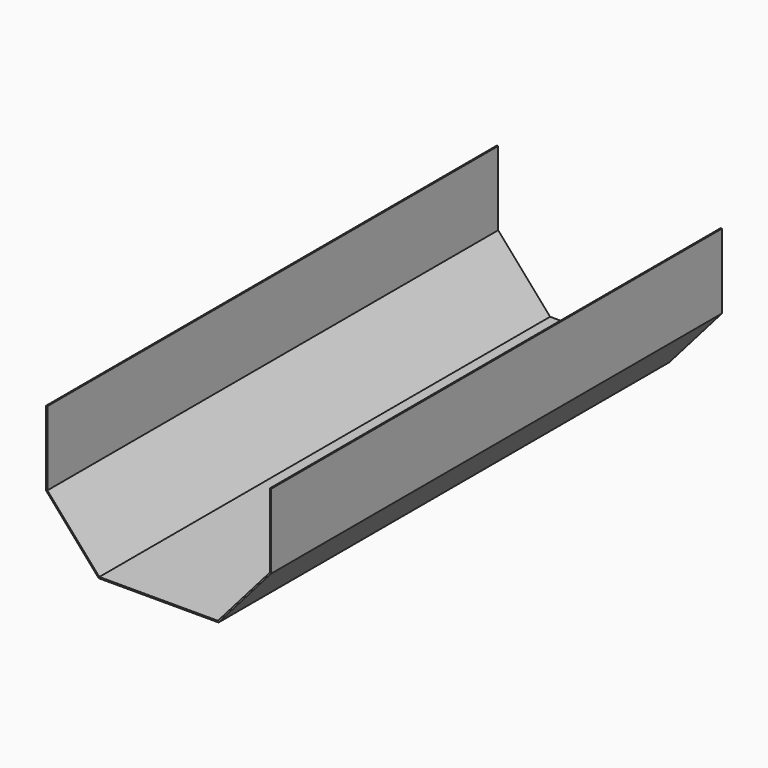
from build123d import *

# Parameters (mm, degrees)
F1_DEPTH = 965.2


# Not quite as in the source:
# - a feature names something its author has since deleted; it is built from what else it names


with BuildPart() as f1:
    # F0 (on Front) → F1 (new body)
    with BuildSketch(Plane.XZ):
        Polygon((-88.9, 101.6), (-88.9, 228.6), (-91.186, 228.6), (-91.186, 100.7410695246), (-1.037314166, -2.286), (204.237314166, -2.286), (294.386, 100.7410695246), (294.386, 228.6), (292.1, 228.6), (292.1, 101.6), (203.2, 0), (0, 0), align=None)
    extrude(amount=F1_DEPTH)


solid = f1.part
